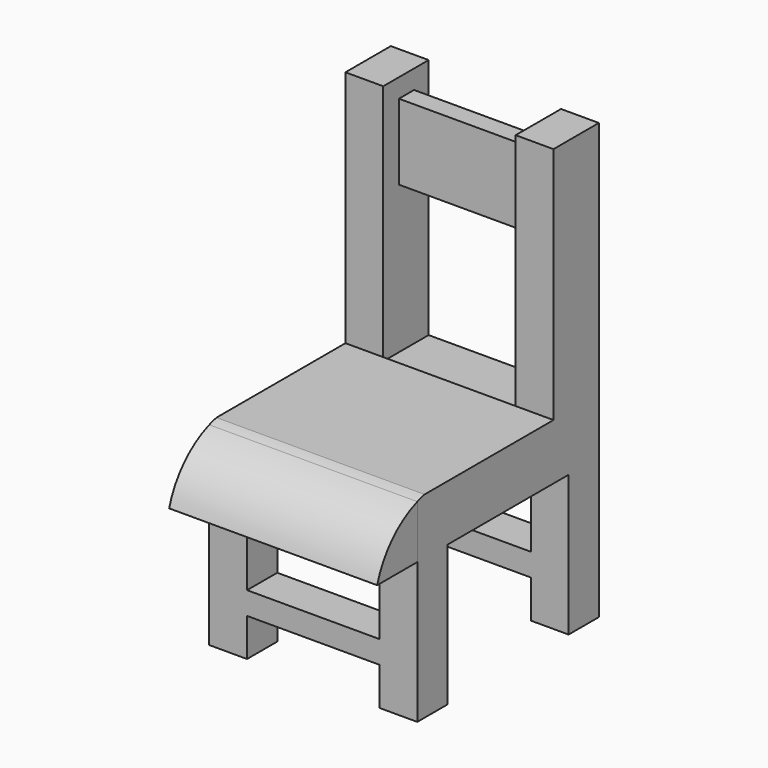
from build123d import *

# Parameters (mm, degrees)
F0_W      = 60
F0_H      = 115
F1_DEPTH  = 55
F2_W      = 35
F2_H      = 10.0414325121
F3_DEPTH  = 90
F2_H_2    = 20.9734155115
F4_DEPTH  = 96
F7_DEPTH  = 55
F9_DEPTH  = 95
F10_W     = 35
F10_H     = 15
F11_DEPTH = 5
F12_W     = 35
F12_H     = 4.8255780712
F12_H_2   = 5.1744219288
F13_DEPTH = 59
F14_W     = 35
F14_H     = 39
F15_DEPTH = 25
F17_DEPTH = 95


with BuildPart() as f1:
    # F0 (on Right) → F1 (new body)
    with BuildSketch(Plane.YZ):
        with Locations((-30, -4.5705132011)):
            Rectangle(F0_W, F0_H)
    extrude(amount=F1_DEPTH)

    # F2 (on face) → F3 (cut)
    with BuildSketch(Plane.XZ.offset(60)):
        with Locations((27.5, -57.049796945)):
            Rectangle(F2_W, F2_H)
    extrude(amount=-F3_DEPTH, mode=Mode.SUBTRACT)

    # F2 (on face) → F4 (cut)
    with BuildSketch(Plane.XZ.offset(60)):
        with Locations((27.5, -35.5572209568)):
            Rectangle(F2_W, F2_H_2)
    extrude(amount=-F4_DEPTH, mode=Mode.SUBTRACT)

    # F8 (on face) → F9 (cut)
    with BuildSketch(Plane(origin=(0, 0, 0), x_dir=(0, -1, 0), z_dir=(-1, 0, 0))):
        with BuildLine():
            Line((15, 52.9294867989), (15, -10.1117771119))
            Line((15, -10.1117771119), (57.598117739, -10.1117771119))
            ThreePointArc((57.598117739, -10.1117771119), (58.8094054709, -10.4277742826), (60, -10.8145000884))
            Line((60, -10.8145000884), (60, 52.9294867989))
            Line((60, 52.9294867989), (15, 52.9294867989))
        make_face()
    extrude(amount=-F9_DEPTH, mode=Mode.SUBTRACT)

    # F10 (on face) → F11 (cut)
    with BuildSketch(Plane.XY.offset(52.9294867989)):
        with Locations((27.5, -7.5)):
            Rectangle(F10_W, F10_H)
    extrude(amount=-F11_DEPTH, mode=Mode.SUBTRACT)

    # F12 (on face) → F13 (cut)
    with BuildSketch(Plane.XY.offset(47.9294867989)):
        with Locations((27.5, -2.4127890356)):
            Rectangle(F12_W, F12_H)
        with Locations((27.5, -12.4127890356)):
            Rectangle(F12_W, F12_H_2)
    extrude(amount=-F13_DEPTH, mode=Mode.SUBTRACT)

    # F14 (on face) → F15 (cut)
    with BuildSketch(Plane.XZ.offset(9.8255780712)):
        with Locations((27.5, 8.4294867989)):
            Rectangle(F14_W, F14_H)
    extrude(amount=-F15_DEPTH, mode=Mode.SUBTRACT)

    # F16 (on face) → F17 (cut)
    with BuildSketch(Plane(origin=(0, 0, 0), x_dir=(0, -1, 0), z_dir=(-1, 0, 0))):
        Polygon((50.0226652549, -62.0705132011), (50.0226652549, -45.8980772977), (50.0226652549, -24.8737987131), (10, -24.8737987131), (10, -45.8980772977), (10, -62.0705132011), align=None)
    extrude(amount=-F17_DEPTH, mode=Mode.SUBTRACT)


with BuildPart() as f7:
    # F6 (on face) → F7 (new body)
    with BuildSketch(Plane(origin=(0, 0, 0), x_dir=(0, -1, 0), z_dir=(-1, 0, 0))):
        with BuildLine():
            ThreePointArc((73.2497498393, -24.8737987131), (68.3136194252, -16.25264453), (60, -10.8145000884))
            Line((60, -10.8145000884), (60, -24.8737987131))
            Line((60, -24.8737987131), (73.2497498393, -24.8737987131))
        make_face()
    extrude(amount=-F7_DEPTH)


solid = Compound([f1.part, f7.part])
